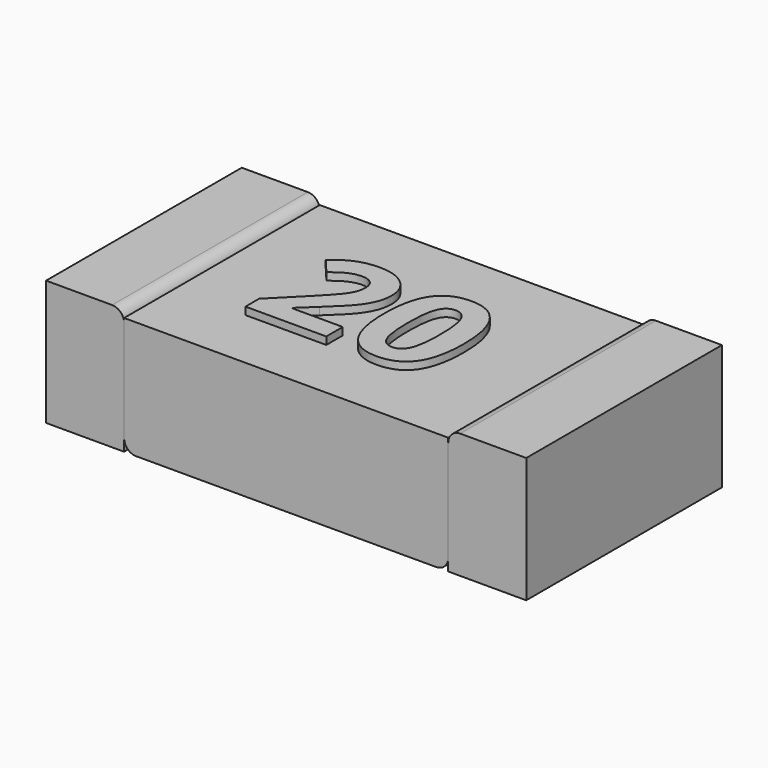
from build123d import *

# Parameters (mm, degrees)
F0_W         = 0.52
F0_H         = 1.63
F1_DEPTH     = 0.835
F0_W_2       = 2.16
F2_DEPTH     = 0.785
F3_TEXT_SIZE = 1.0792506348
F4_DEPTH     = 0.05
F5_R         = 0.08
F5_2_R       = 0.08
F5_3_R       = 0.08


# Not quite as in the source:
# - Text() gives the source's letters only with a copy of the font that has no kerning and outlines rounded to 1/6400 em; it was checked with that copy


with BuildPart() as f1:
    # F0 (on Top) → F1 (new body)
    with BuildSketch(Plane.XY):
        with Locations((-1.34, 0)):
            Rectangle(F0_W, F0_H)
    extrude(amount=F1_DEPTH)

    # F5#2
    f5_2_edges = [f1.edges().sort_by_distance(p)[0] for p in [
        (-1.08, 0, 0.835),
    ]]
    fillet(f5_2_edges, radius=F5_2_R)


with BuildPart() as f1b:
    # F0 (on Top) → F1, piece 2 (new body)
    with BuildSketch(Plane.XY):
        with Locations((1.34, 0)):
            Rectangle(F0_W, F0_H)
    extrude(amount=F1_DEPTH)

    # F5
    f5_edges = [f1b.edges().sort_by_distance(p)[0] for p in [
        (1.08, 0, 0.835),
    ]]
    fillet(f5_edges, radius=F5_R)


with BuildPart() as f2:
    # F0 (on Top) → F2 (new body)
    with BuildSketch(Plane.XY):
        Rectangle(F0_W_2, F0_H)
    extrude(amount=F2_DEPTH)

    # F5#3
    f5_3_edges = [f2.edges().sort_by_distance(p)[0] for p in [
        (-1.08, 0, 0),
        (1.08, 0, 0),
    ]]
    fillet(f5_3_edges, radius=F5_3_R)


with BuildPart() as f4:
    # F3 (on face) → F4 (new body)
    with BuildSketch(Plane.XY.offset(0.785)):
        with Locations((-0.6500828822, -0.3954110725)):
            Text('20', F3_TEXT_SIZE, font='Open Sans', font_style=FontStyle.BOLD, text_align=(TextAlign.LEFT, TextAlign.BOTTOM))
    extrude(amount=F4_DEPTH)


solid = Compound([f1.part, f1b.part, f2.part, f4.part])
